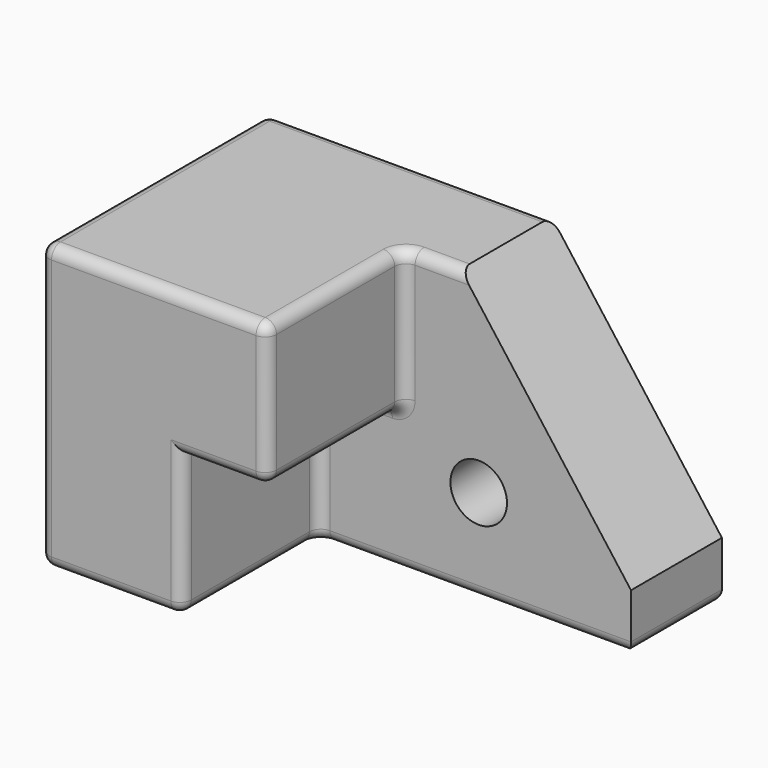
from build123d import *

# Parameters (mm, degrees)
F0_W     = 203.2
F0_H     = 127
F1_DEPTH = 127
F3_DEPTH = 76.2
F4_SIZE2 = 101.6
F4_SIZE  = 76.2
F5_R     = 5.08
F6_R     = 12.6476198181
F7_DEPTH = 78.486


with BuildPart() as f1:
    # F0 (on Front) → F1 (new body)
    with BuildSketch(Plane.XZ):
        Rectangle(F0_W, F0_H)
    extrude(amount=F1_DEPTH)

    # F2 (on face) → F3 (cut)
    with BuildSketch(Plane.XZ.offset(127)):
        Polygon((101.6, 63.5), (0, 63.5), (0, 0), (-38.1, 0), (-38.1, -63.5), (101.6, -63.5), align=None)
    extrude(amount=-F3_DEPTH, mode=Mode.SUBTRACT)

    # F4
    f4_edges = [f1.edges().sort_by_distance(p)[0] for p in [
        (101.6, -25.4, 63.5),
    ]]
    f4_side = f1.faces().sort_by_distance((-21.771429, -52.614286, 63.5))[0]
    chamfer(f4_edges, length=F4_SIZE, length2=F4_SIZE2, reference=f4_side)

    # F5
    f5_edges = [f1.edges().sort_by_distance(p)[0] for p in [
        (0, -88.9, 63.5),
        (-50.8, -127, 63.5),
        (-19.05, -127, 0),
        (0, -127, 31.75),
        (0, -88.9, 0),
        (-38.1, -127, -31.75),
        (-38.1, -88.9, -63.5),
        (-69.85, -127, -63.5),
        (0, -50.8, 31.75),
        (31.75, -50.8, -63.5),
        (-38.1, -50.8, -31.75),
        (0, 0, -63.5),
        (-38.1, 0, 63.5),
        (-101.6, -127, 0),
        (-101.6, -63.5, 63.5),
        (-101.6, 0, 0),
        (101.6, -25.4, -63.5),
        (-101.6, -63.5, -63.5),
        (12.7, -50.8, 63.5),
        (-19.05, -50.8, 0),
    ]]
    fillet(f5_edges, radius=F5_R)

    # F6 (on face) → F7 (cut)
    with BuildSketch(Plane.XZ.offset(50.8)):
        with Locations((33.5065871477, -21.8299999833)):
            Circle(F6_R)
    extrude(amount=-F7_DEPTH, mode=Mode.SUBTRACT)


solid = f1.part
